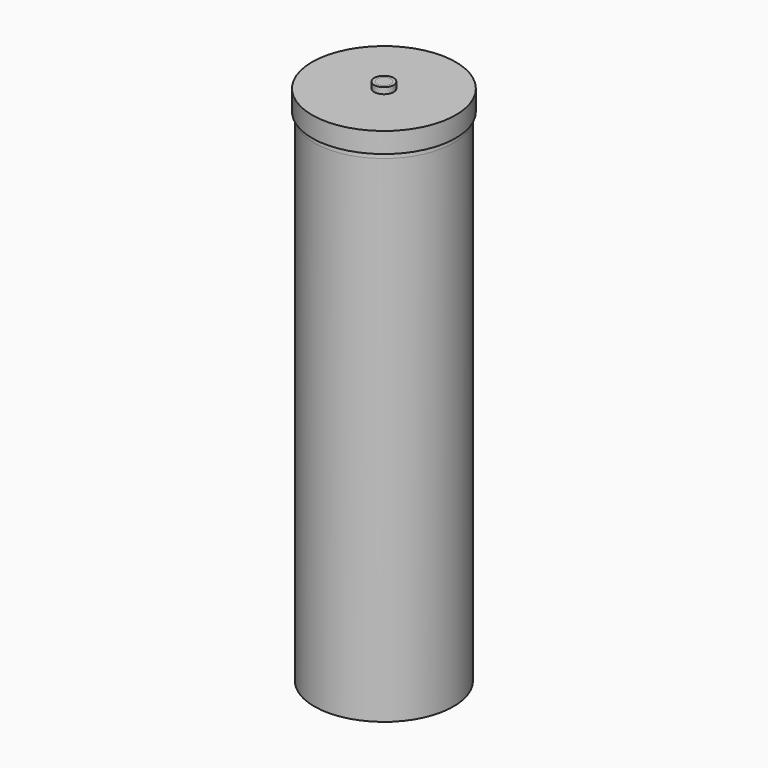
from build123d import *

# Parameters (mm, degrees)
F3_T          = -3.175
F4_T          = -4.7625
F6_DEPTH      = 50.0136
F6_DEPTH_BACK = 50.0136
F7_W          = 40.0304
F7_H          = 3.175
F11_R         = 6.985
F11_R_2       = 3.81
F12_DEPTH     = 4.445
F13_R         = 4.9276
F14_DEPTH     = 25.4
F15_R         = 6.985
F15_R_2       = 3.81
F16_DEPTH     = 4.445
F18_R         = 4.4196
F19_DEPTH     = 3.175
F20_W         = 12.7
F20_H         = 3.175
F21_DEPTH     = 28.575
F22_R         = 4.8895
F22_W         = 12.7
F22_H         = 3.175
F23_DEPTH     = 3.175
F24_W         = 4.9276
F24_H         = 8.89
F24_H_2       = 3.81
F29_R         = 15.875
F29_R_2       = 14.224
F30_DEPTH     = 79.756


# Not quite as in the source:
# - a length typed as a fraction of an inch, garbled in the dataset ("3 / 203.2 mm" for 3/8 in), is restored


with BuildPart() as f1:
    # F0 (on Front) → F1 (revolve)
    with BuildSketch(Plane.XZ):
        with BuildLine():
            ThreePointArc((0, 30.9626), (-35.364249, 16.314249), (-50.0126, -19.05))
            Line((-50.0126, -19.05), (-50.0126, -375.4374))
            Line((-50.0126, -375.4374), (0, -375.4374))
            Line((0, -375.4374), (0, 30.9626))
        make_face()
    revolve(axis=Axis((0, 0, -172.2374), (0, 0, -1)))

    # F3
    f3_openings = [f1.faces().sort_by_distance(p)[0] for p in [
        (0, 0, -375.4374),
    ]]
    offset(amount=F3_T, openings=f3_openings)


with BuildPart() as f2:
    # F0 (on Front) → F2 (revolve)
    with BuildSketch(Plane.XZ):
        with BuildLine():
            ThreePointArc((0, 30.9626), (-35.364249, 16.314249), (-50.0126, -19.05))
            Line((-50.0126, -19.05), (-50.0126, -375.4374))
            Line((-50.0126, -375.4374), (0, -375.4374))
            Line((0, -375.4374), (0, 30.9626))
        make_face()
    revolve(axis=Axis((0, 0, -172.2374), (0, 0, -1)))

    # F4
    f4_openings = [f2.faces().sort_by_distance(p)[0] for p in [
        (0, 0, -375.4374),
    ]]
    offset(amount=F4_T, openings=f4_openings)


with BuildPart() as f6_tool:
    # F5 (on Front) → F6 (new body, two sides)
    with BuildSketch(Plane.XZ) as f6_sk:
        with BuildLine():
            ThreePointArc((46.864926, -1.5875), (0, 30.9626), (-46.864926, -1.5875))
            Line((-46.864926, -1.5875), (46.864926, -1.5875))
        make_face()
    extrude(amount=-F6_DEPTH)
    extrude(f6_sk.sketch, amount=F6_DEPTH_BACK)


with BuildPart() as f1_1:
    add(f1.part)

    # F6: cut by f6_tool
    add(f6_tool.part, mode=Mode.SUBTRACT)


with BuildPart() as f2_1:
    add(f2.part)

    # F6: cut by f6_tool
    add(f6_tool.part, mode=Mode.SUBTRACT)


with BuildPart() as f8:
    # F7 (on Front) → F8 (revolve)
    with BuildSketch(Plane.XZ):
        Polygon((-51.6001, -0.8255), (-51.6001, -15.4305), (-50.8381, -15.4305), (-50.8381, -1.5875), (-4.4196, -1.5875), (-4.4196, -0.8255), align=None)
    revolve(axis=Axis((0, 0, -187.7187), (0, 0, -1)))


with BuildPart() as f9:
    # F7 (on Front) → F9 (revolve)
    with BuildSketch(Plane.XZ):
        with Locations((-24.4348, -5.87409)):
            Rectangle(F7_W, F7_H)
    revolve(axis=Axis((0, 0, -187.7187), (0, 0, -1)))


with BuildPart() as f12:
    # F11 (on offset) → F12 (new body)
    with BuildSketch(Plane.XY.offset(3.6195)):
        Circle(F11_R)
        Circle(F11_R_2, mode=Mode.SUBTRACT)
    extrude(amount=-F12_DEPTH)


with BuildPart() as f14:
    # F13 (on face) → F14 (new body)
    with BuildSketch(Plane.XY.offset(3.6195)):
        Circle(F13_R)
    extrude(amount=-F14_DEPTH)


with BuildPart() as f16:
    # F15 (on face) → F16 (new body)
    with BuildSketch(Plane(origin=(0, 0, -7.46159), x_dir=(1, 0, 0), z_dir=(0, 0, -1))):
        Circle(F15_R)
        Circle(F15_R_2, mode=Mode.SUBTRACT)
    extrude(amount=F16_DEPTH)


with BuildPart() as f19:
    # F18 (on offset) → F19 (new body)
    with BuildSketch(Plane(origin=(0, 0, -15.71659), x_dir=(1, 0, 0), z_dir=(0, 0, -1))):
        with BuildLine():
            Line((6.35, -13.97), (6.35, -7.269017))
            ThreePointArc((6.35, -7.269017), (0, 9.652), (-6.35, -7.269017))
            Line((-6.35, -7.269017), (-6.35, -13.97))
            Line((-6.35, -13.97), (6.35, -13.97))
        make_face()
        Circle(F18_R, mode=Mode.SUBTRACT)
    extrude(amount=F19_DEPTH)

    # F20 (on face) → F21 (join)
    with BuildSketch(Plane(origin=(0, 0, -18.89159), x_dir=(1, 0, 0), z_dir=(0, 0, -1))):
        with Locations((0, -12.3825)):
            Rectangle(F20_W, F20_H)
    extrude(amount=F21_DEPTH)

    # F22 (on face) → F23 (join)
    with BuildSketch(Plane(origin=(0, 0, -47.46659), x_dir=(1, 0, 0), z_dir=(0, 0, -1))):
        with BuildLine():
            ThreePointArc((6.35, -7.269017), (0, 9.652), (-6.35, -7.269017))
            Line((-6.35, -7.269017), (-6.35, -10.795))
            Line((-6.35, -10.795), (6.35, -10.795))
            Line((6.35, -10.795), (6.35, -7.269017))
        make_face()
        Circle(F22_R, mode=Mode.SUBTRACT)
        with Locations((0, -12.3825)):
            Rectangle(F22_W, F22_H)
    extrude(amount=-F23_DEPTH)


with BuildPart() as f25_1:
    # F25: copy of F9
    add(f9.part.moved(Location((0, 0, -6.4008))))


with BuildPart() as f26:
    # F24 (on Front) → F26 (revolve)
    with BuildSketch(Plane.XZ):
        with Locations((-2.4638, -46.19659)):
            Rectangle(F24_W, F24_H)
        with Locations((-2.4638, -52.54659)):
            Rectangle(F24_W, F24_H_2)
    revolve(axis=Axis((0, 0, -65.24659), (0, 0, -1)))


with BuildPart() as f27:
    # F24 (on Front) → F27 (revolve)
    with BuildSketch(Plane.XZ):
        with Locations((-2.4638, -52.54659)):
            Rectangle(F24_W, F24_H_2)
        Polygon((-4.9276, -54.45159), (-4.9276, -50.64159), (-12.7, -50.64159), (-12.7, -84.67759), (-12.7, -88.74159), (0, -88.74159), (0, -54.45159), align=None)
    revolve(axis=Axis((0, 0, -65.24659), (0, 0, -1)))


with BuildPart() as f28:
    # F24 (on Front) → F28 (revolve)
    with BuildSketch(Plane.XZ):
        Polygon((-12.7, -88.74159), (-12.7, -84.67759), (-14.224, -84.67759), (-14.224, -87.21759), (-18.288, -87.21759), (-18.288, -88.74159), align=None)
    revolve(axis=Axis((0, 0, -65.24659), (0, 0, -1)))


with BuildPart() as f30:
    # F29 (on face) → F30 (new body, through all)
    with BuildSketch(Plane.XY.offset(-87.21759)):
        Circle(F29_R)
        Circle(F29_R_2, mode=Mode.SUBTRACT)
    extrude(amount=F30_DEPTH)


solid = Compound([f1_1.part, f2_1.part, f8.part, f9.part, f12.part, f14.part, f16.part, f19.part, f25_1.part, f26.part, f27.part, f28.part, f30.part])
